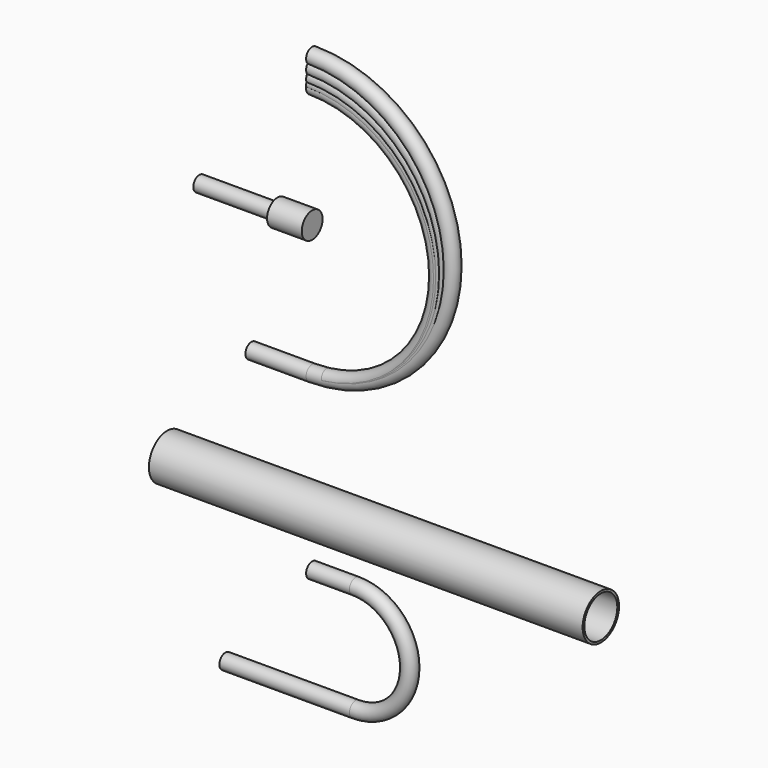
from build123d import *

# Parameters (mm, degrees)
F1_R      = 3
F1_R_2    = 1.75
F1_R_3    = 5.25
F1_R_4    = 4.75
F10_DEPTH = 100
F13_DEPTH = 100


with BuildPart() as f2:
    # F2: sweep along a path in F0
    with BuildLine(Plane.XZ) as f2_path:
        Line((0, 30), (-8, 30))
    # F1 (on Right) → F2 (sweep)
    with BuildSketch(Plane.YZ):
        with Locations((0, 30)):
            Circle(F1_R)
        with Locations((0, 30)):
            Circle(F1_R_2, mode=Mode.SUBTRACT)
    sweep(path=f2_path.line)

    # F3: sweep along a path in F0
    with BuildLine(Plane.XZ) as f3_path:
        Line((-26, 30), (-8, 30))
        Line((-8, 30), (0, 30))
    # F1 (on Right) → F3 (sweep)
    with BuildSketch(Plane.YZ):
        with Locations((0, 30)):
            Circle(F1_R_2)
    sweep(path=f3_path.line)


with BuildPart() as f4:
    # F4: sweep along a path in F0
    with BuildLine(Plane.XZ) as f4_path:
        Line((0, 0), (-14, 0))
    # F1 (on Right) → F4 (sweep)
    with BuildSketch(Plane.YZ):
        Circle(F1_R_2)
    sweep(path=f4_path.line)


with BuildPart() as f5:
    # F5: sweep along a path in F0
    with BuildLine(Plane.XZ) as f5_path:
        ThreePointArc((0, 0), (31.1, 31.1), (0, 62.2))
    # F1 (on Right) → F5 (sweep)
    with BuildSketch(Plane.YZ):
        Circle(F1_R_2)
    sweep(path=f5_path.line)


with BuildPart() as f6:
    # F6: sweep along a path in F0
    with BuildLine(Plane.XZ) as f6_path:
        ThreePointArc((0, 0), (29.55, 29.55), (0, 59.1))
    # F1 (on Right) → F6 (sweep)
    with BuildSketch(Plane.YZ):
        Circle(F1_R_2)
    sweep(path=f6_path.line)


with BuildPart() as f7:
    # F7: sweep along a path in F0
    with BuildLine(Plane.XZ) as f7_path:
        ThreePointArc((0, 0), (29.2, 29.2), (0, 58.4))
    # F1 (on Right) → F7 (sweep)
    with BuildSketch(Plane.YZ):
        Circle(F1_R_2)
    sweep(path=f7_path.line)


with BuildPart() as f8:
    # F8: sweep along a path in F0
    with BuildLine(Plane.XZ) as f8_path:
        ThreePointArc((0, 0), (30.15, 30.15), (0, 60.3))
    # F1 (on Right) → F8 (sweep)
    with BuildSketch(Plane.YZ):
        Circle(F1_R_2)
    sweep(path=f8_path.line)


with BuildPart() as f9:
    # F9: sweep along a path in F0
    with BuildLine(Plane.XZ) as f9_path:
        ThreePointArc((0, 0), (32.225, 32.225), (0, 64.45))
    # F1 (on Right) → F9 (sweep)
    with BuildSketch(Plane.YZ):
        Circle(F1_R_2)
    sweep(path=f9_path.line)


with BuildPart() as f10:
    # F1 (on Right) → F10 (new body)
    with BuildSketch(Plane.YZ):
        with Locations((-41.8023914099, 0)):
            Circle(F1_R_3)
        with Locations((-41.8023914099, 0)):
            Circle(F1_R_4, mode=Mode.SUBTRACT)
    extrude(amount=F10_DEPTH)


with BuildPart() as f11:
    # F11: sweep along a path in F0
    with BuildLine(Plane.XZ) as f11_path:
        Line((0, -40), (10, -40))
        ThreePointArc((10, -40), (22.5, -52.5), (10, -65))
        Line((10, -65), (-20, -65))
    # F1 (on Right) → F11 (sweep)
    with BuildSketch(Plane.YZ):
        with Locations((0, -40)):
            Circle(F1_R_2)
    sweep(path=f11_path.line)


with BuildPart() as f12:
    # F12: sweep along a path in F0
    with BuildLine(Plane.XZ) as f12_path:
        Line((0, -40), (10, -40))
        ThreePointArc((10, -40), (22.5, -52.5), (10, -65))
        Line((10, -65), (-20, -65))
    # F1 (on Right) → F12 (sweep)
    with BuildSketch(Plane.YZ):
        with Locations((0, -40)):
            Circle(F1_R_2)
    sweep(path=f12_path.line)


with BuildPart() as f13:
    # F1 (on Right) → F13 (new body)
    with BuildSketch(Plane.YZ):
        with Locations((-41.8023914099, 0)):
            Circle(F1_R_3)
        with Locations((-41.8023914099, 0)):
            Circle(F1_R_4, mode=Mode.SUBTRACT)
    extrude(amount=F13_DEPTH)


solid = Compound([f2.part, f4.part, f5.part, f6.part, f7.part, f8.part, f9.part, f10.part, f11.part, f12.part, f13.part])
